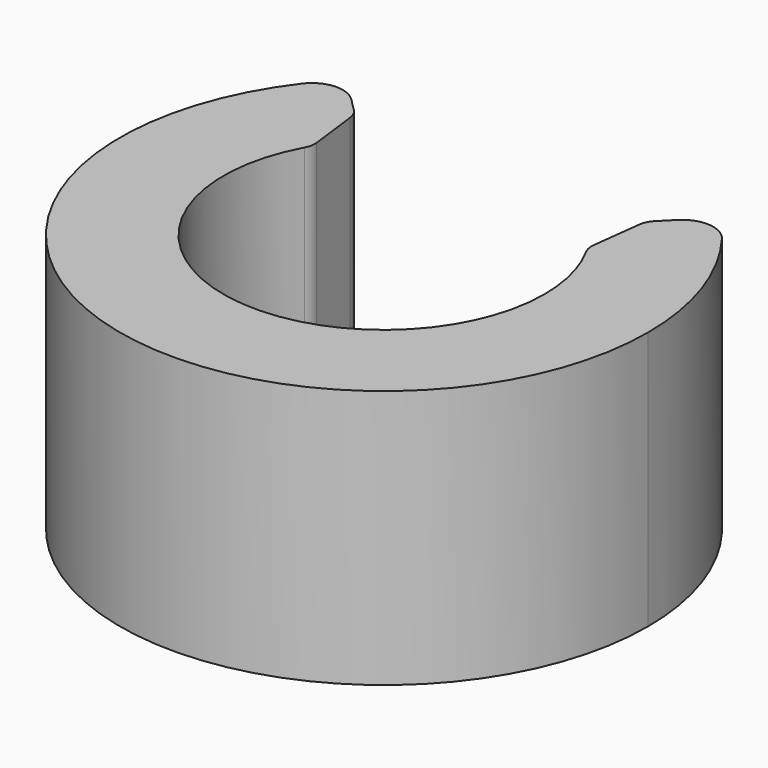
from build123d import *

# Parameters (mm, degrees)
F1_DEPTH    = 25
F2_R        = 3
F3_T1_DEPTH = 47.7014436638
F4_R        = 2


# Not quite as in the source:
# - a fillet or chamfer that OpenCascade refuses, or shapes differently, is made with other operations: its cross-section is extruded or revolved along the edge and cut away or added


with BuildPart() as f1:
    # F0 (on Top) → F1 (new body)
    with BuildSketch(Plane.XY):
        with BuildLine():
            ThreePointArc((10.9601551084, 10.9601551084), (14.3201327539, 5.9315932017), (15.5, 0))
            ThreePointArc((15.5, 0), (-5.9315932017, -14.3201327539), (-10.9601551084, 10.9601551084))
            Line((-10.9601551084, 10.9601551084), (-18.0312229203, 18.0312229203))
            ThreePointArc((-18.0312229203, 18.0312229203), (-9.7584275253, -23.558928079), (25.5, 0))
            ThreePointArc((25.5, 0), (23.558928079, 9.7584275253), (18.0312229203, 18.0312229203))
            Line((18.0312229203, 18.0312229203), (10.9601551084, 10.9601551084))
        make_face()
    extrude(amount=F1_DEPTH)

    # F2
    f2_edges = [f1.edges().sort_by_distance(p)[0] for p in [
        (-18.031223, 18.031223, 12.5),
        (18.031223, 18.031223, 12.5),
    ]]
    fillet(f2_edges, radius=F2_R)

    # F3: chamfer of 5 on 2 edges, made by hand

    # F3_s2 → F3_t1 (cut)
    with BuildSketch(Plane.XY.offset(-11.3507218319)):
        with BuildLine():
            Line((-14.0579159195, 14.0579159195), (-13.3023645022, 7.9559473761))
            ThreePointArc((-13.3023645022, 7.9559473761), (-12.2677824681, 9.4737275301), (-10.9601551084, 10.9601551084))
            Line((-10.9601551084, 10.9601551084), (-14.0579159195, 14.0579159195))
        make_face()
        with BuildLine():
            Line((13.3023645022, 7.9559473761), (14.0579159195, 14.0579159195))
            Line((14.0579159195, 14.0579159195), (10.9601551084, 10.9601551084))
            ThreePointArc((10.9601551084, 10.9601551084), (12.2677824681, 9.4737275301), (13.3023645022, 7.9559473761))
        make_face()
    extrude(amount=F3_T1_DEPTH, mode=Mode.SUBTRACT)

    # F4
    f4_edges = [f1.edges().sort_by_distance(p)[0] for p in [
        (-13.302365, 7.955947, 12.5),
        (-14.057916, 14.057916, 12.5),
        (13.302365, 7.955947, 12.5),
        (14.057916, 14.057916, 12.5),
    ]]
    fillet(f4_edges, radius=F4_R)


solid = f1.part
